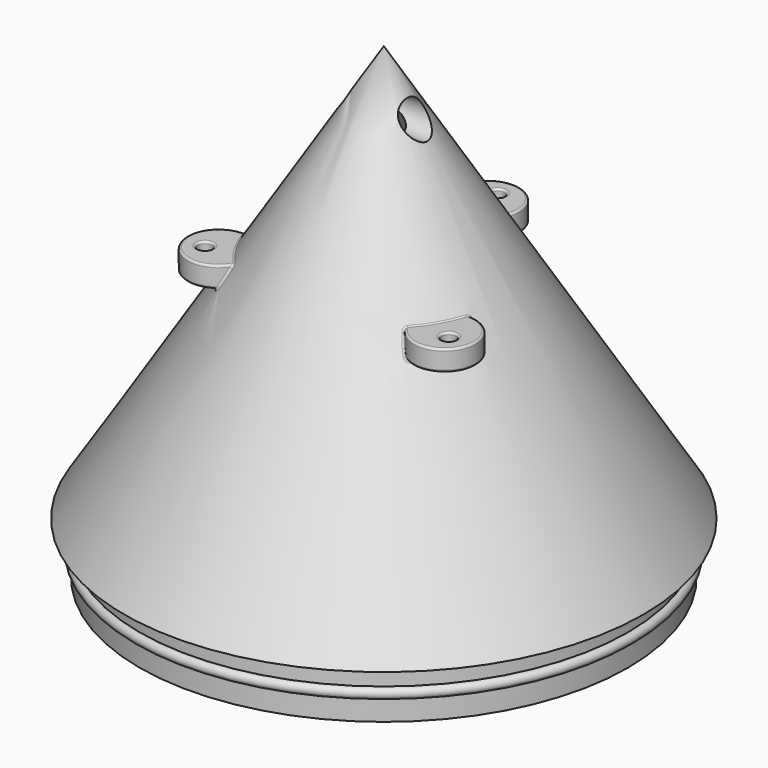
from build123d import *

# Parameters (mm, degrees)
F2_T           = -2.54
F3_R           = 29.845
F3_R_2         = 28.7547109906
F4_DEPTH       = 6.35
F7_R           = 0.635
F9_R           = 1.9447019749
F10_DEPTH      = 31.751
F10_DEPTH_BACK = 31.751
F14_DEPTH      = 2.54
F16_R          = 0.889
F17_DEPTH      = 2.54
F18_R          = 0.254


with BuildPart() as f1:
    # F0 (on Front) → F1 (revolve)
    with BuildSketch(Plane.XZ):
        Polygon((31.75, 0), (0, 50.8), (0, 0), align=None)
    revolve(axis=Axis((0, 0, 25.4), (0, 0, -1)))

    # F2
    f2_openings = [f1.faces().sort_by_distance(p)[0] for p in [
        (0, 0, 0),
    ]]
    offset(amount=F2_T, openings=f2_openings)

    # F3 (on face) → F4 (join)
    with BuildSketch(Plane(origin=(0, 0, 0), x_dir=(1, 0, 0), z_dir=(0, 0, -1))):
        Circle(F3_R)
        Circle(F3_R_2, mode=Mode.SUBTRACT)
    extrude(amount=F4_DEPTH)

    # F8: sweep along a path in F6
    with BuildLine(Plane(origin=(0, 0, -3.175), x_dir=(1, 0, 0), z_dir=(0, 0, -1))) as f8_path:
        CenterArc((0, 0), 29.845, 0, 360)
    # F7 (on Right) → F8 (sweep)
    with BuildSketch(Plane.YZ):
        with Locations((-29.8586767167, -3.175)):
            Circle(F7_R)
    sweep(path=f8_path.line)

    # F9 (on Right) → F10 (cut, two sides)
    with BuildSketch(Plane.YZ) as f10_sk:
        with Locations((0, 44.2378930748)):
            Circle(F9_R)
    extrude(amount=-F10_DEPTH, mode=Mode.SUBTRACT)
    extrude(f10_sk.sketch, amount=F10_DEPTH_BACK, mode=Mode.SUBTRACT)

    # F13 (on offset) → F14 (join)
    with BuildSketch(Plane.XY.offset(25.4)):
        with BuildLine():
            ThreePointArc((-10.2907916393, -9.44777791), (-12.0983748909, -6.985), (-13.327411499, -4.1881980297))
            ThreePointArc((-13.327411499, -4.1881980297), (-17.1014653906, -9.8735356468), (-10.2907916393, -9.44777791))
        make_face()
        with BuildLine():
            ThreePointArc((0, 13.97), (1.5274678593, 13.8862429022), (3.0366198597, 13.6359759397))
            ThreePointArc((3.0366198597, 13.6359759397), (0, 19.7470712936), (-3.0366198597, 13.6359759397))
            ThreePointArc((-3.0366198597, 13.6359759397), (-1.5274678593, 13.8862429022), (0, 13.97))
        make_face()
        with BuildLine():
            ThreePointArc((13.327411499, -4.1881980297), (12.0983748909, -6.985), (10.2907916393, -9.44777791))
            ThreePointArc((10.2907916393, -9.44777791), (17.1014653906, -9.8735356468), (13.327411499, -4.1881980297))
        make_face()
    extrude(amount=F14_DEPTH)

    # F16 (on offset) → F17 (cut, through all)
    with BuildSketch(Plane.XY.offset(27.94)):
        with Locations((0, 17.3427684085)):
            Circle(F16_R)
        with Locations((14.9078106989, -8.7223370816)):
            Circle(F16_R)
        with Locations((-14.9920785309, -8.5766873165)):
            Circle(F16_R)
    extrude(amount=-F17_DEPTH, mode=Mode.SUBTRACT)

    # F18
    f18_edges = [f1.edges().sort_by_distance(p)[0] for p in [
        (-13.748153, -7.9375, 25.4),
        (-10.891665, -10.427516, 26.674385),
        (-14.476326, -4.218701, 26.674385),
        (-12.373338, -7.14375, 27.94),
        (-17.101465, -9.873536, 27.94),
        (-17.101465, -9.873536, 25.4),
        (17.101465, -9.873536, 27.94),
        (17.101465, -9.873536, 25.4),
        (12.373338, -7.14375, 27.94),
        (0, 14.2875, 27.94),
        (-3.584661, 14.646217, 26.674385),
        (3.584661, 14.646217, 26.674385),
        (0, 19.747071, 27.94),
        (0, 19.747071, 25.4),
        (-0.889, 17.342768, 27.94),
        (-15.881079, -8.576687, 27.94),
        (14.018811, -8.722337, 27.94),
        (14.477968, -4.218996, 26.67173),
        (13.748153, -7.9375, 25.4),
        (10.892742, -10.42879, 26.67173),
        (0, 15.875, 25.4),
    ]]
    fillet(f18_edges, radius=F18_R)


solid = f1.part
